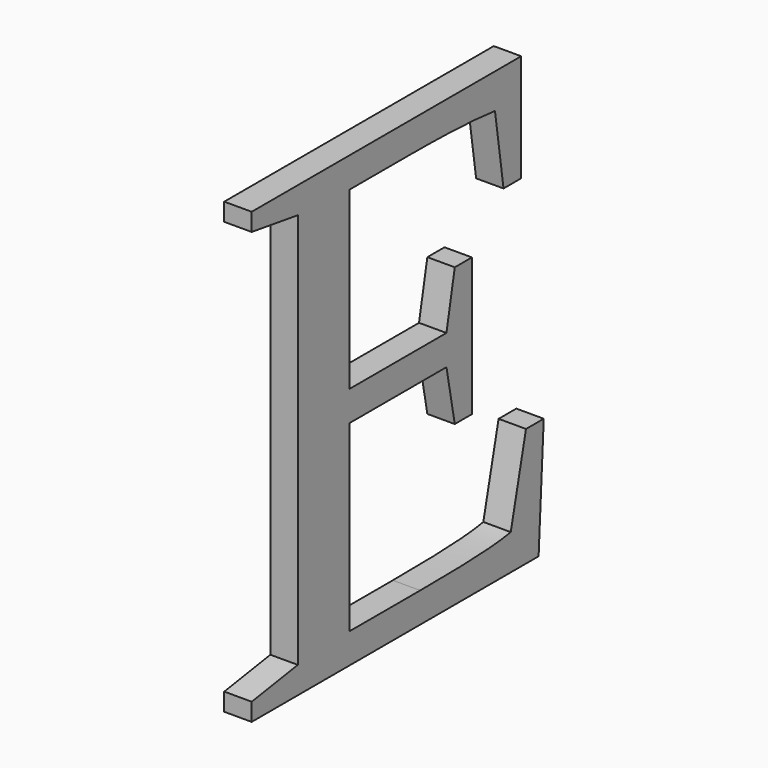
from build123d import *

# Parameters (mm, degrees)
F0_TEXT_SIZE = 635
F1_DEPTH     = 25.4


# Not quite as in the source:
# - Text() gives the source's letters only with a copy of the font that has no kerning and outlines rounded to 1/6400 em; it was checked with that copy


with BuildPart() as f1:
    # F0 (on Right) → F1 (new body)
    with BuildSketch(Plane.YZ):
        with Locations((-508.1671011149, 0)):
            Text('E', F0_TEXT_SIZE, font='Tinos', text_align=(TextAlign.LEFT, TextAlign.BOTTOM))
    extrude(amount=F1_DEPTH)


solid = f1.part
